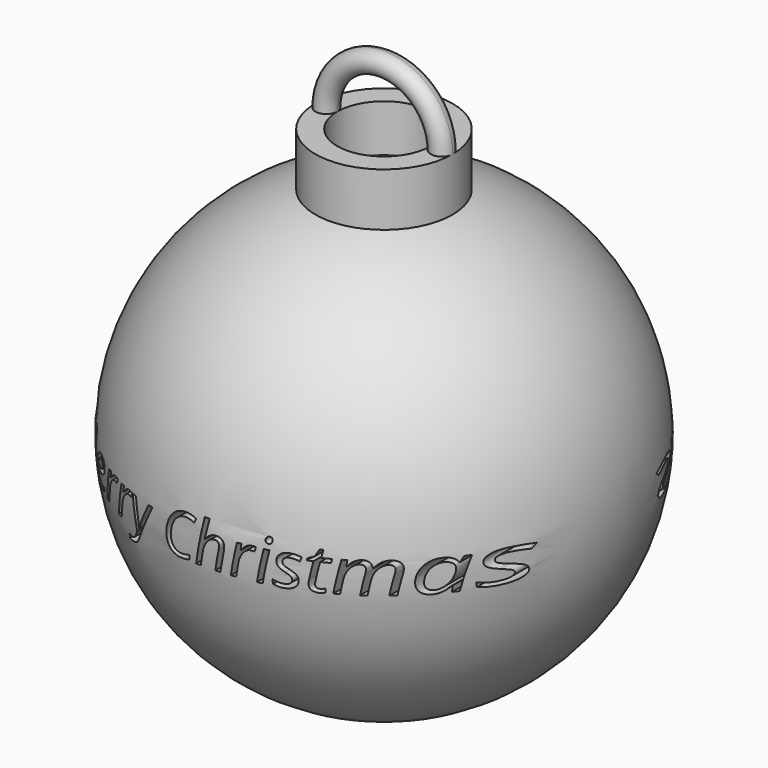
from build123d import *

# Parameters (mm, degrees)
F2_R         = 17.1668749166
F2_R_2       = 11.6922225939
F3_DEPTH     = 67.056
F7_TEXT_SIZE = 14.5988666788
F8_DEPTH     = 137.414


# Not quite as in the source:
# - Text() gives the source's letters only with a copy of the font that has no kerning and outlines rounded to 1/6400 em; it was checked with that copy


with BuildPart() as f1:
    # F0 (on Front) → F1 (revolve)
    with BuildSketch(Plane.XZ):
        with BuildLine():
            Line((0, -56.4276223298), (0, 56.4276223298))
            ThreePointArc((0, 56.4276223298), (-56.4276223298, 0), (0, -56.4276223298))
        make_face()
    revolve(axis=Axis((0, 0, -0.7164105773), (0, 0, -1)))

    # F7 (on Front) → F8 (cut, symmetric)
    with BuildSketch(Plane.XZ):
        with Locations((-52.6686629912, -6.6165741439)):
            Text('Merry Christmas', F7_TEXT_SIZE, font='Open Sans', font_style=FontStyle.ITALIC, text_align=(TextAlign.LEFT, TextAlign.BOTTOM))
    extrude(amount=F8_DEPTH, both=True, mode=Mode.SUBTRACT)


with BuildPart() as f3:
    # F2 (on Top) → F3 (new body)
    with BuildSketch(Plane.XY):
        Circle(F2_R)
        Circle(F2_R_2, mode=Mode.SUBTRACT)
    extrude(amount=F3_DEPTH)


with BuildPart() as f6:
    # F6: sweep along a path in F5
    with BuildLine(Plane.XZ) as f6_path:
        ThreePointArc((14.4295487553, 67.056), (0, 81.4855487553), (-14.4295487553, 67.056))
    # F4 (on face) → F6 (sweep)
    with BuildSketch(Plane.XY.offset(67.056)):
        with BuildLine():
            ThreePointArc((11.6922225939, 0), (14.4295487553, -2.7373261614), (17.1668749166, 0))
            ThreePointArc((17.1668749166, 0), (14.4295487553, 2.7373261614), (11.6922225939, 0))
        make_face()
    sweep(path=f6_path.line)


solid = Compound([f1.part, f3.part, f6.part])
